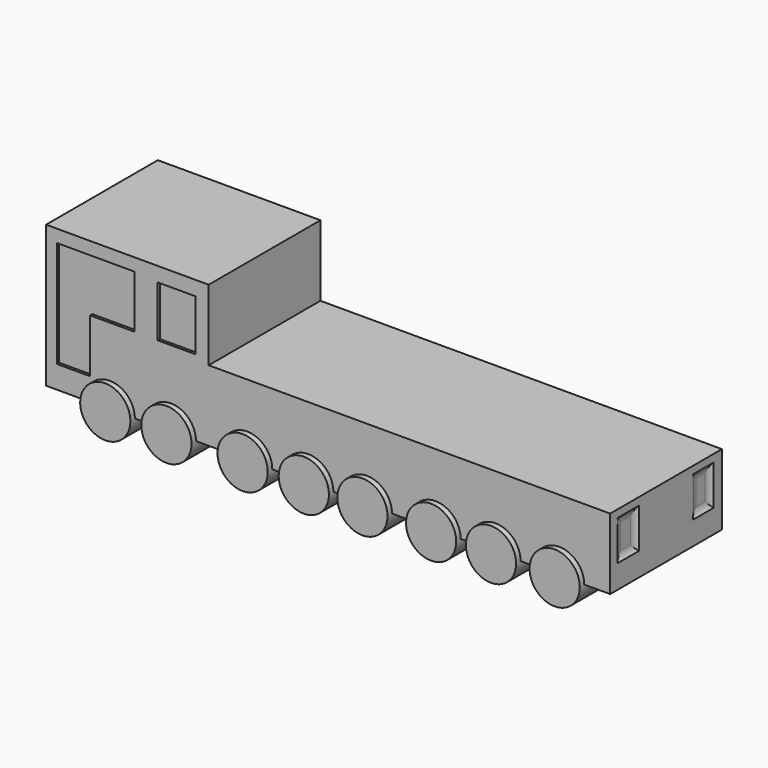
from build123d import *

# Parameters (mm, degrees)
F0_W         = 17.1937867999
F0_H         = 23.2116123661
F1_DEPTH     = 31.75
F2_W         = 8.8453050703
F2_H         = 5.5423062295
F2_H_2       = 5.7832766324
F2_W_2       = 53.1131848693
F2_H_3       = 7.2131637233
F3_DEPTH     = 1.27
F2_H_4       = 29.5187777961
F4_DEPTH     = 1.27
F5_T1_DEPTH  = 14.1835370451
F5_T6_DEPTH  = 22.3428270547
F5_T11_DEPTH = 22.3428270547
F6_R         = 1.26999
F7_DEPTH     = 34.29
F0_W_2       = 15.1878371835
F0_H_2       = 24.3578637019
F8_DEPTH     = 30.48
F9_W         = 12.2006889433
F9_H         = 18.1582923979
F9_W_2       = 11.8028419092
F10_DEPTH    = 1.27
F11_T1_DEPTH = 26.5585528105
F11_T3_DEPTH = 20.6009493559
F11_T5_DEPTH = 20.2031023219


# Not quite as in the source:
# - a fillet or chamfer that OpenCascade refuses, or shapes differently, is made with other operations: its cross-section is extruded or revolved along the edge and cut away or added
# - a fillet or chamfer is up to 0.001 mm smaller than in the source, because OpenCascade refuses the exact size


with BuildPart() as f1:
    # F0 (on Front) → F1 (new body, symmetric)
    with BuildSketch(Plane.XZ):
        with BuildLine():
            Line((-58.7454400957, 35.6771033257), (-132.6787173748, 35.6771033257))
            Line((-132.6787173748, 35.6771033257), (-132.6787173748, -28.7995953113))
            Line((-132.6787173748, -28.7995953113), (-115.1552961537, -28.7995953113))
            ThreePointArc((-115.1552961537, -28.7995953113), (-103.7358418107, -17.3801409683), (-92.3163874677, -28.7995953113))
            Line((-92.3163874677, -28.7995953113), (-87.3586775133, -28.7995953113))
            ThreePointArc((-87.3586775133, -28.7995953113), (-75.9392231703, -17.3801409683), (-64.5197688273, -28.7995953113))
            Line((-64.5197688273, -28.7995953113), (-58.7454400957, -28.7995953113))
            Line((-58.7454400957, -28.7995953113), (-58.7454400957, 3.4387540072))
            Line((-58.7454400957, 3.4387540072), (-58.7454400957, 35.6771033257))
        make_face()
        Polygon((-127.8071403503, 5.8745397255), (-127.8071403503, 29.9458410591), (-92.5598889589, 29.9458410591), (-92.5598889589, 5.8745397255), (-112.6193031669, 5.8745397255), (-112.6193031669, -18.4833239764), (-127.8071403503, -18.4833239764), align=None, mode=Mode.SUBTRACT)
        with Locations((-73.3601562679, 17.4803459086)):
            Rectangle(F0_W, F0_H, mode=Mode.SUBTRACT)
        with BuildLine():
            Line((123.7952634692, 3.4387540072), (-58.7454400957, 3.4387540072))
            Line((-58.7454400957, 3.4387540072), (-58.7454400957, -28.7995953113))
            Line((-58.7454400957, -28.7995953113), (-52.6845434078, -28.7995953113))
            ThreePointArc((-52.6845434078, -28.7995953113), (-41.2650890648, -17.3801409683), (-29.8456347218, -28.7995953113))
            Line((-29.8456347218, -28.7995953113), (-24.8879229048, -28.7995953113))
            ThreePointArc((-24.8879229048, -28.7995953113), (-13.4684685618, -17.3801409683), (-2.0490142188, -28.7995953113))
            Line((-2.0490142188, -28.7995953113), (1.7624453312, -28.7995953113))
            ThreePointArc((1.7624453312, -28.7995953113), (13.1818996742, -17.3801409683), (24.6013540172, -28.7995953113))
            Line((24.6013540172, -28.7995953113), (32.9978263608, -28.7995953113))
            ThreePointArc((32.9978263608, -28.7995953113), (44.4172807038, -17.3801409683), (55.8367350468, -28.7995953113))
            Line((55.8367350468, -28.7995953113), (60.2213128141, -28.7995953113))
            ThreePointArc((60.2213128141, -28.7995953113), (71.6407671571, -17.3801409683), (83.0602215001, -28.7995953113))
            Line((83.0602215001, -28.7995953113), (89.1641883782, -28.7995953113))
            ThreePointArc((89.1641883782, -28.7995953113), (100.5836427212, -17.3801409683), (112.0030970642, -28.7995953113))
            Line((112.0030970642, -28.7995953113), (123.7952634692, -28.7995953113))
            Line((123.7952634692, -28.7995953113), (123.7952634692, 3.4387540072))
        make_face()
    extrude(amount=F1_DEPTH, both=True)

    # F2 (on face) → F3 (join)
    with BuildSketch(Plane(origin=(-132.6787173748, 0, 0), x_dir=(0, -1, 0), z_dir=(-1, 0, 0))):
        with Locations((-21.9635469839, -19.9353238568)):
            Rectangle(F2_W, F2_H)
        with Locations((22.3043328151, -20.0558090582)):
            Rectangle(F2_W, F2_H_2)
        with Locations((0.1703929156, -8.744909234)):
            Rectangle(F2_W_2, F2_H_3)
    extrude(amount=F3_DEPTH)

    # F2 (on face) → F4 (cut)
    with BuildSketch(Plane(origin=(-132.6787173748, 0, 0), x_dir=(0, -1, 0), z_dir=(-1, 0, 0))):
        with Locations((0.1703929156, 14.759388898)):
            Rectangle(F2_W_2, F2_H_4)
    extrude(amount=-F4_DEPTH, mode=Mode.SUBTRACT)

    # F5: fillet of radius 5.08 on 4 edges, made by hand

    # F5_s2 → F5_t1 (cut)
    with BuildSketch(Plane.XY.offset(-31.3477077871)):
        with BuildLine():
            ThreePointArc((-132.6787173748, -26.7269853503), (-133.620622256, -25.1629324094), (-133.9487173748, -23.3668811852))
            Line((-133.9487173748, -23.3668811852), (-133.9487173748, -26.7269853503))
            Line((-133.9487173748, -26.7269853503), (-132.6787173748, -26.7269853503))
        make_face()
        with BuildLine():
            ThreePointArc((-132.6787173748, -17.88168028), (-133.620622256, -19.4457332208), (-133.9487173748, -21.241784445))
            Line((-133.9487173748, -21.241784445), (-133.9487173748, -17.88168028))
            Line((-133.9487173748, -17.88168028), (-132.6787173748, -17.88168028))
        make_face()
    extrude(amount=F5_T1_DEPTH, mode=Mode.SUBTRACT)


with BuildPart() as f5_tool4:
    # F5_s5 → F5_t6 (new body)
    with BuildSketch(Plane.XY.offset(-31.1067373841)):
        with BuildLine():
            ThreePointArc((-132.6787173748, 17.5408944488), (-133.620622256, 19.1049473896), (-133.9487173748, 20.9009986138))
            Line((-133.9487173748, 20.9009986138), (-133.9487173748, 17.5408944488))
            Line((-133.9487173748, 17.5408944488), (-132.6787173748, 17.5408944488))
        make_face()
    extrude(amount=F5_T6_DEPTH)

    split(bisect_by=Plane.XY.offset(-12.3514910956), keep=Keep.BOTTOM)


with BuildPart() as f1_1:
    add(f1.part)

    # F5_t3: cut F5_tool4
    add(f5_tool4.part, mode=Mode.SUBTRACT)


with BuildPart() as f5_tool9:
    # F5_s10 → F5_t11 (new body)
    with BuildSketch(Plane.XY.offset(-8.7639103294)):
        with BuildLine():
            ThreePointArc((-132.6787173748, 26.386199519), (-133.620622256, 24.8221465782), (-133.9487173748, 23.026095354))
            Line((-133.9487173748, 23.026095354), (-133.9487173748, 26.386199519))
            Line((-133.9487173748, 26.386199519), (-132.6787173748, 26.386199519))
        make_face()
    extrude(amount=-F5_T11_DEPTH)

    split(bisect_by=Plane.XY.offset(-12.3514910956), keep=Keep.BOTTOM)


with BuildPart() as f1_2:
    add(f1_1.part)

    # F5_t8: cut F5_tool9
    add(f5_tool9.part, mode=Mode.SUBTRACT)

    # F6 (radius 1.27 in the source; OpenCascade refuses exactly that, so slightly less here)
    f6_edges = [f1_2.edges().sort_by_distance(p)[0] for p in [
        (-133.948717, -0.170393, -12.351491),
        (-133.948717, 26.3862, -8.744909),
        (-133.948717, -0.170393, -5.138327),
        (-133.948717, -26.726985, -8.744909),
    ]]
    fillet(f6_edges, radius=F6_R)

    # F0 (on Front) → F8 (join, symmetric)
    with BuildSketch(Plane.XZ):
        Polygon((-92.5598889589, 29.9458410591), (-127.8071403503, 29.9458410591), (-127.8071403503, 5.8745397255), (-112.6193031669, 5.8745397255), (-92.5598889589, 5.8745397255), align=None)
        with Locations((-120.2132217586, -6.3043921255)):
            Rectangle(F0_W_2, F0_H_2)
        with Locations((-73.3601562679, 17.4803459086)):
            Rectangle(F0_W, F0_H)
    extrude(amount=F8_DEPTH, both=True)

    # F9 (on face) → F10 (cut)
    with BuildSketch(Plane.YZ.offset(123.7952634692)):
        with Locations((-21.4970195666, -9.0791461989)):
            Rectangle(F9_W, F9_H)
        with Locations((21.1390811019, -9.0791461989)):
            Rectangle(F9_W_2, F9_H)
    extrude(amount=-F10_DEPTH, mode=Mode.SUBTRACT)

    # F11: fillet of radius 5.08 on 8 edges, made by hand

    # F11_s2 → F11_t1 (join)
    with BuildSketch(Plane.XY.offset(-26.5585528105)):
        with BuildLine():
            ThreePointArc((123.7952634692, -27.5973640382), (122.853358588, -26.0333110974), (122.5252634692, -24.2372598732))
            Line((122.5252634692, -24.2372598732), (122.5252634692, -27.5973640382))
            Line((122.5252634692, -27.5973640382), (123.7952634692, -27.5973640382))
        make_face()
        with BuildLine():
            ThreePointArc((123.7952634692, -15.396675095), (122.853358588, -16.9607280358), (122.5252634692, -18.75677926))
            Line((122.5252634692, -18.75677926), (122.5252634692, -15.396675095))
            Line((122.5252634692, -15.396675095), (123.7952634692, -15.396675095))
        make_face()
        with BuildLine():
            ThreePointArc((123.7952634692, 15.2376601472), (122.853358588, 16.8017130881), (122.5252634692, 18.5977643123))
            Line((122.5252634692, 18.5977643123), (122.5252634692, 15.2376601472))
            Line((122.5252634692, 15.2376601472), (123.7952634692, 15.2376601472))
        make_face()
        with BuildLine():
            ThreePointArc((123.7952634692, 27.0405020565), (122.853358588, 25.4764491156), (122.5252634692, 23.6803978914))
            Line((122.5252634692, 23.6803978914), (122.5252634692, 27.0405020565))
            Line((122.5252634692, 27.0405020565), (123.7952634692, 27.0405020565))
        make_face()
    extrude(amount=F11_T1_DEPTH)

    # F11_s4 → F11_t3 (join)
    with BuildSketch(Plane.XZ.offset(6.9964146823)):
        with BuildLine():
            ThreePointArc((123.7952634692, 0), (122.853358588, -1.5640529408), (122.5252634692, -3.3601041651))
            Line((122.5252634692, -3.3601041651), (122.5252634692, 0))
            Line((122.5252634692, 0), (123.7952634692, 0))
        make_face()
        with BuildLine():
            ThreePointArc((123.7952634692, -18.1582923979), (122.853358588, -16.594239457), (122.5252634692, -14.7981882328))
            Line((122.5252634692, -14.7981882328), (122.5252634692, -18.1582923979))
            Line((122.5252634692, -18.1582923979), (123.7952634692, -18.1582923979))
        make_face()
    extrude(amount=F11_T3_DEPTH)

    # F11_s6 → F11_t5 (join)
    with BuildSketch(Plane.XZ.offset(-27.0405020565)):
        with BuildLine():
            ThreePointArc((123.7952634692, 0), (122.853358588, -1.5640529408), (122.5252634692, -3.3601041651))
            Line((122.5252634692, -3.3601041651), (122.5252634692, 0))
            Line((122.5252634692, 0), (123.7952634692, 0))
        make_face()
        with BuildLine():
            ThreePointArc((123.7952634692, -18.1582923979), (122.853358588, -16.594239457), (122.5252634692, -14.7981882328))
            Line((122.5252634692, -14.7981882328), (122.5252634692, -18.1582923979))
            Line((122.5252634692, -18.1582923979), (123.7952634692, -18.1582923979))
        make_face()
    extrude(amount=F11_T5_DEPTH)


with BuildPart() as f7:
    # F0 (on Front) → F7 (new body, symmetric)
    with BuildSketch(Plane.XZ):
        with BuildLine():
            ThreePointArc((-92.3163874677, -28.7995953113), (-103.7358418107, -17.3801409683), (-115.1552961537, -28.7995953113))
            ThreePointArc((-115.1552961537, -28.7995953113), (-103.7358418107, -40.2190496543), (-92.3163874677, -28.7995953113))
        make_face()
    extrude(amount=F7_DEPTH, both=True)


with BuildPart() as f7b:
    # F0 (on Front) → F7, piece 2 (new body, symmetric)
    with BuildSketch(Plane.XZ):
        with BuildLine():
            ThreePointArc((-87.3586775133, -28.7995953113), (-75.9392231703, -40.2190496543), (-64.5197688273, -28.7995953113))
            ThreePointArc((-64.5197688273, -28.7995953113), (-75.9392231703, -17.3801409683), (-87.3586775133, -28.7995953113))
        make_face()
    extrude(amount=F7_DEPTH, both=True)


with BuildPart() as f7c:
    # F0 (on Front) → F7, piece 3 (new body, symmetric)
    with BuildSketch(Plane.XZ):
        with BuildLine():
            ThreePointArc((-29.8456347218, -28.7995953113), (-41.2650890648, -17.3801409683), (-52.6845434078, -28.7995953113))
            ThreePointArc((-52.6845434078, -28.7995953113), (-41.2650890648, -40.2190496543), (-29.8456347218, -28.7995953113))
        make_face()
    extrude(amount=F7_DEPTH, both=True)


with BuildPart() as f7d:
    # F0 (on Front) → F7, piece 4 (new body, symmetric)
    with BuildSketch(Plane.XZ):
        with BuildLine():
            ThreePointArc((-2.0490142188, -28.7995953113), (-13.4684685618, -17.3801409683), (-24.8879229048, -28.7995953113))
            ThreePointArc((-24.8879229048, -28.7995953113), (-13.4684685618, -40.2190496543), (-2.0490142188, -28.7995953113))
        make_face()
    extrude(amount=F7_DEPTH, both=True)


with BuildPart() as f7e:
    # F0 (on Front) → F7, piece 5 (new body, symmetric)
    with BuildSketch(Plane.XZ):
        with BuildLine():
            ThreePointArc((24.6013540172, -28.7995953113), (13.1818996742, -17.3801409683), (1.7624453312, -28.7995953113))
            ThreePointArc((1.7624453312, -28.7995953113), (13.1818996742, -40.2190496543), (24.6013540172, -28.7995953113))
        make_face()
    extrude(amount=F7_DEPTH, both=True)


with BuildPart() as f7f:
    # F0 (on Front) → F7, piece 6 (new body, symmetric)
    with BuildSketch(Plane.XZ):
        with BuildLine():
            ThreePointArc((32.9978263608, -28.7995953113), (44.4172807038, -40.2190496543), (55.8367350468, -28.7995953113))
            ThreePointArc((55.8367350468, -28.7995953113), (44.4172807038, -17.3801409683), (32.9978263608, -28.7995953113))
        make_face()
    extrude(amount=F7_DEPTH, both=True)


with BuildPart() as f7g:
    # F0 (on Front) → F7, piece 7 (new body, symmetric)
    with BuildSketch(Plane.XZ):
        with BuildLine():
            ThreePointArc((60.2213128141, -28.7995953113), (71.6407671571, -40.2190496543), (83.0602215001, -28.7995953113))
            ThreePointArc((83.0602215001, -28.7995953113), (71.6407671571, -17.3801409683), (60.2213128141, -28.7995953113))
        make_face()
    extrude(amount=F7_DEPTH, both=True)


with BuildPart() as f7h:
    # F0 (on Front) → F7, piece 8 (new body, symmetric)
    with BuildSketch(Plane.XZ):
        with BuildLine():
            ThreePointArc((89.1641883782, -28.7995953113), (100.5836427212, -40.2190496543), (112.0030970642, -28.7995953113))
            ThreePointArc((112.0030970642, -28.7995953113), (100.5836427212, -17.3801409683), (89.1641883782, -28.7995953113))
        make_face()
    extrude(amount=F7_DEPTH, both=True)


solid = Compound([f1_2.part, f7.part, f7b.part, f7c.part, f7d.part, f7e.part, f7f.part, f7g.part, f7h.part])
